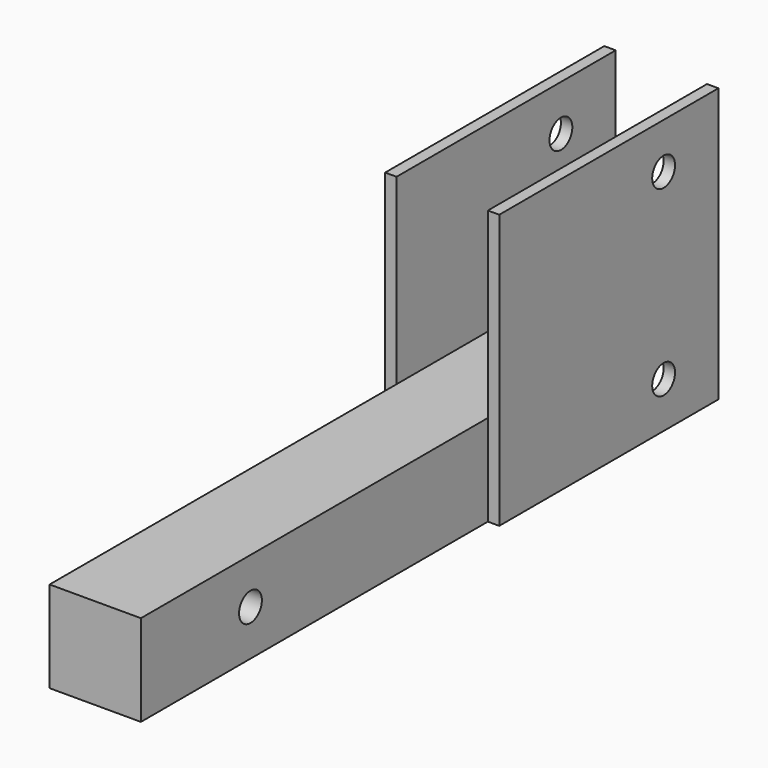
from build123d import *

# Parameters (mm, degrees)
F0_W      = 50.8
F0_H      = 304.8
F1_DEPTH  = 50.8
F2_W      = 63.5
F2_H      = 50.8
F3_DEPTH  = 6.35
F4_R      = 7.94131
F4_R_2    = 7.9375
F5_DEPTH  = 6.35
F6_R      = 7.9375
F7_DEPTH  = 50.8
F8_W      = 63.5
F8_H      = 50.8
F9_DEPTH  = 6.35
F10_R     = 7.9375
F11_DEPTH = 6.35


with BuildPart() as f1:
    # F0 (on Top) → F1 (new body)
    with BuildSketch(Plane.XY):
        with Locations((-25.4, -152.4)):
            Rectangle(F0_W, F0_H)
    extrude(amount=F1_DEPTH)

    # F2 (on face) → F3 (join)
    with BuildSketch(Plane(origin=(-50.8, 0, 0), x_dir=(0, -1, 0), z_dir=(-1, 0, 0))):
        Polygon((-88.9, 0), (0, 0), (0, 50.8), (63.5, 50.8), (63.5, 152.4), (-88.9, 152.4), align=None)
        with Locations((31.75, 25.4)):
            Rectangle(F2_W, F2_H)
    extrude(amount=F3_DEPTH)

    # F4 (on face) → F5 (cut)
    with BuildSketch(Plane(origin=(-57.15, 0, 0), x_dir=(0, -1, 0), z_dir=(-1, 0, 0))):
        with Locations((-50.8, 127)):
            Circle(F4_R)
        with Locations((-50.8, 25.4)):
            Circle(F4_R_2)
    extrude(amount=-F5_DEPTH, mode=Mode.SUBTRACT)

    # F6 (on face) → F7 (cut)
    with BuildSketch(Plane(origin=(-50.8, 0, 0), x_dir=(0, -1, 0), z_dir=(-1, 0, 0))):
        with Locations((228.6, 25.4)):
            Circle(F6_R)
    extrude(amount=-F7_DEPTH, mode=Mode.SUBTRACT)

    # F8 (on face) → F9 (join)
    with BuildSketch(Plane.YZ):
        with Locations((-31.75, 25.4)):
            Rectangle(F8_W, F8_H)
        Polygon((0, 50.8), (0, 0), (88.9, 0), (88.9, 152.4), (-63.5, 152.4), (-63.5, 50.8), align=None)
    extrude(amount=F9_DEPTH)

    # F10 (on face) → F11 (cut)
    with BuildSketch(Plane.YZ.offset(6.35)):
        with Locations((50.8, 127)):
            Circle(F10_R)
        with Locations((50.8, 25.4)):
            Circle(F10_R)
    extrude(amount=-F11_DEPTH, mode=Mode.SUBTRACT)


solid = f1.part
